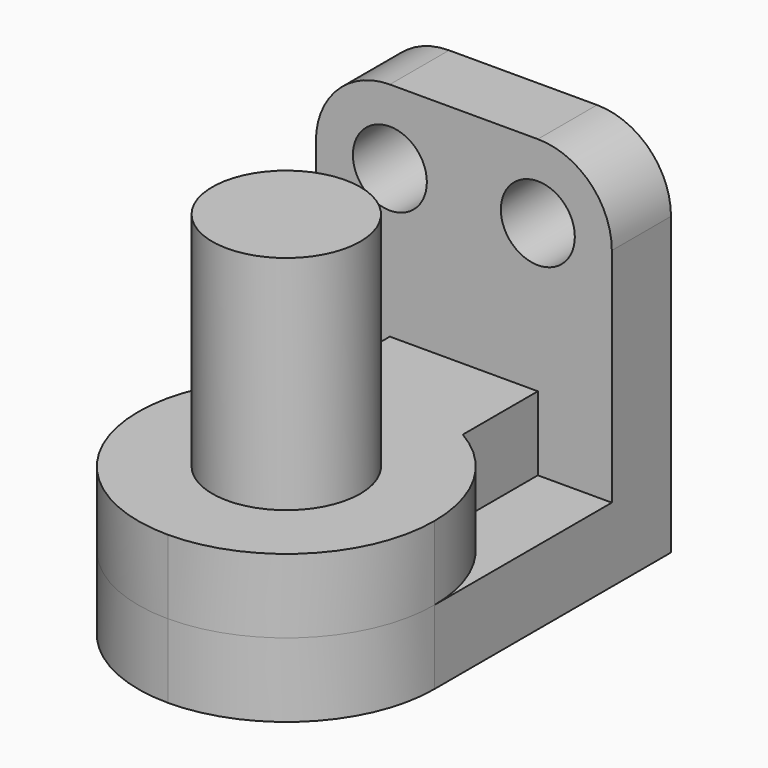
from build123d import *

# Parameters (mm, degrees)
F1_DEPTH = 20
F2_R     = 19.99999
F3_R     = 10
F5_DEPTH = 10
F6_R     = 10
F7_DEPTH = 30
F9_D     = 10
F9_DEPTH = 10.001


# Not quite as in the source:
# - a fillet or chamfer is up to 0.001 mm smaller than in the source, because OpenCascade refuses the exact size


with BuildPart() as f1:
    # F0 (on Right) → F1 (new body, symmetric)
    with BuildSketch(Plane.YZ):
        Polygon((-60, 0), (0, 0), (0, 50), (-10, 50), (-10, 10), (-60, 10), align=None)
    extrude(amount=F1_DEPTH, both=True)

    # F2 (radius 20 in the source; OpenCascade refuses exactly that, so slightly less here)
    f2_edges = [f1.edges().sort_by_distance(p)[0] for p in [
        (-20, -60, 5),
        (20, -60, 5),
    ]]
    fillet(f2_edges, radius=F2_R)

    # F3
    f3_edges = [f1.edges().sort_by_distance(p)[0] for p in [
        (-20, -5, 50),
        (20, -5, 50),
    ]]
    fillet(f3_edges, radius=F3_R)

    # F4 (on face) → F5 (join)
    with BuildSketch(Plane.XY.offset(10)):
        with BuildLine():
            Line((-10, -10), (-10, -22.6794919243))
            ThreePointArc((-10, -22.6794919243), (-17.3205105757, -30.0000043301), (-20, -40.00001))
            ThreePointArc((-20, -40.00001), (-14.1421320882, -54.1421391593), (0, -60))
            ThreePointArc((0, -60), (14.1421320882, -54.1421391593), (20, -40.00001))
            ThreePointArc((20, -40.00001), (17.3205105757, -30.0000043301), (10, -22.6794919243))
            Line((10, -22.6794919243), (10, -10))
            Line((10, -10), (-10, -10))
        make_face()
    extrude(amount=F5_DEPTH)

    # F6 (on face) → F7 (join)
    with BuildSketch(Plane.XY.offset(20)):
        with Locations((0, -40)):
            Circle(F6_R)
    extrude(amount=F7_DEPTH)

    # F9 (through all, one way)
    with BuildSketch(Plane.XZ.offset(10)):
        with Locations((10, 40), (-10, 40)):
            Circle(F9_D / 2)
    extrude(amount=-F9_DEPTH, mode=Mode.SUBTRACT)


solid = f1.part
